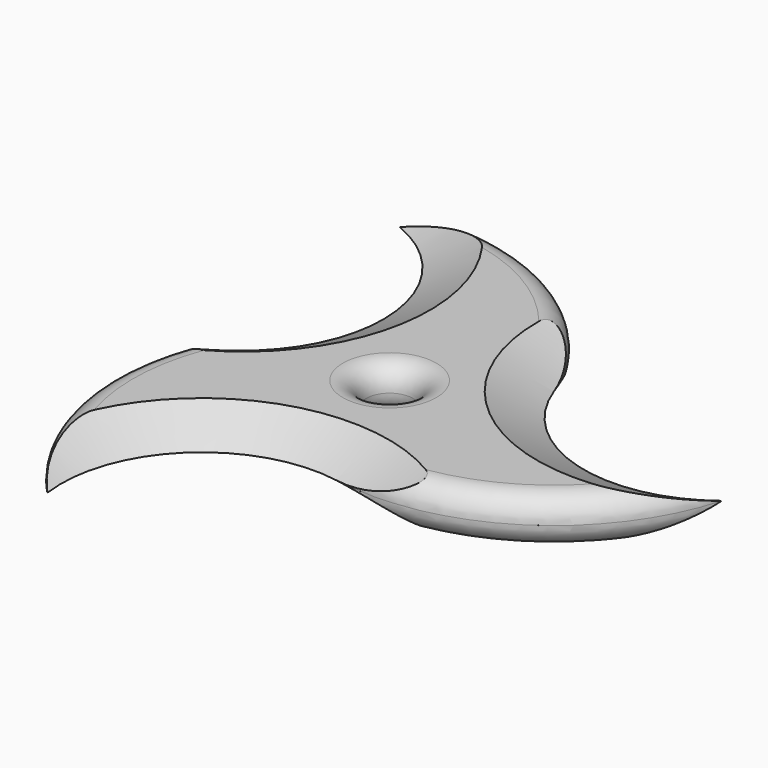
from build123d import *

# Parameters (mm, degrees)
F0_R        = 3.175
F1_DEPTH    = 3.175
F2_T2_ANGLE = 206.8397195509
F2_T4_ANGLE = 206.8397195509
F2_T6_ANGLE = 206.8397195509
F3_R        = 3.17499


# Not quite as in the source:
# - a fillet or chamfer that OpenCascade refuses, or shapes differently, is made with other operations: its cross-section is extruded or revolved along the edge and cut away or added
# - a fillet or chamfer is up to 0.001 mm smaller than in the source, because OpenCascade refuses the exact size


with BuildPart() as f1:
    # F0 (on Top) → F1 (new body)
    with BuildSketch(Plane.XY):
        with BuildLine():
            Line((6.1187519112, -16.6939891892), (-17.516794684, 3.048))
            ThreePointArc((-17.516794684, 3.048), (-24.6567837547, -17.812740491), (-16.0209838859, -38.1))
            ThreePointArc((-16.0209838859, -38.1), (-10.3962463249, -21.7652237747), (6.1187519112, -16.6939891892))
        make_face()
        with BuildLine():
            ThreePointArc((41.0060598271, 5.1754209612), (24.0473598704, 1.879198466), (11.3980427727, 13.6459891892))
            Line((11.3980427727, 13.6459891892), (6.1187519112, -16.6939891892))
            ThreePointArc((6.1187519112, -16.6939891892), (27.7546776535, -12.4470308617), (41.0060598271, 5.1754209612))
        make_face()
        with BuildLine():
            ThreePointArc((-24.9850759412, 32.9245790388), (-13.6511135455, 19.8860253087), (-17.516794684, 3.048))
            Line((-17.516794684, 3.048), (11.3980427727, 13.6459891892))
            ThreePointArc((11.3980427727, 13.6459891892), (-3.0978938988, 30.2597713527), (-24.9850759412, 32.9245790388))
        make_face()
        Polygon((11.3980427727, 13.6459891892), (-17.516794684, 3.048), (6.1187519112, -16.6939891892), align=None)
        Circle(F0_R, mode=Mode.SUBTRACT)
    extrude(amount=F1_DEPTH)

    # F2: chamfer of 3.175 x 6.35 on 3 edges, made by hand

    # F2_s1 → F2_t2 (revolve, cut)
    with BuildSketch(Plane(origin=(0.9537550873, 21.4539943341, 0), x_dir=(0, 0, 1), z_dir=(0.0444119638, 0.999013302, 0))):
        Polygon((0, 47.4113941081), (3.175, 53.7613941081), (3.175, 47.4113941081), align=None)
    revolve(axis=Axis((29.2871650632, 20.1944091266, 3.175), (0, 0, -1)), revolution_arc=F2_T2_ANGLE, mode=Mode.SUBTRACT)

    # F2_s3 → F2_t4 (revolve, cut)
    with BuildSketch(Plane(origin=(-19.0565816496, -9.9010210324, 0), x_dir=(0, 0, 1), z_dir=(-0.8873768801, -0.4610447621, 0))):
        Polygon((0, 47.4113941081), (3.175, 53.7613941081), (3.175, 47.4113941081), align=None)
    revolve(axis=Axis((-32.1324538496, 15.2662243863, 3.175), (0, 0, -1)), revolution_arc=F2_T4_ANGLE, mode=Mode.SUBTRACT)

    # F2_s5 → F2_t6 (revolve, cut)
    with BuildSketch(Plane(origin=(18.1028265623, -11.5529733017, 0), x_dir=(0, 0, 1), z_dir=(0.8429649163, -0.5379685398, 0))):
        Polygon((0, 47.4113941081), (3.175, 53.7613941081), (3.175, 47.4113941081), align=None)
    revolve(axis=Axis((2.8452887864, -35.4606335128, 3.175), (0, 0, -1)), revolution_arc=F2_T6_ANGLE, mode=Mode.SUBTRACT)

    # F3 (radius 3.175 in the source; OpenCascade refuses exactly that, so slightly less here)
    f3_edges = [f1.edges().sort_by_distance(p)[0] for p in [
        (-4.399333, 30.910473, 3.175),
        (28.968921, -11.645302, 3.175),
        (-24.569588, -19.26517, 3.175),
        (-3.175, 0, 3.175),
    ]]
    fillet(f3_edges, radius=F3_R)


with BuildPart() as f4_1:
    # F4: instance of F1
    add(f1.part.mirror(Plane(origin=(0, 0, 0), x_dir=(1, 0, 0), z_dir=(0, 0, -1))))


solid = Compound([f1.part, f4_1.part])
